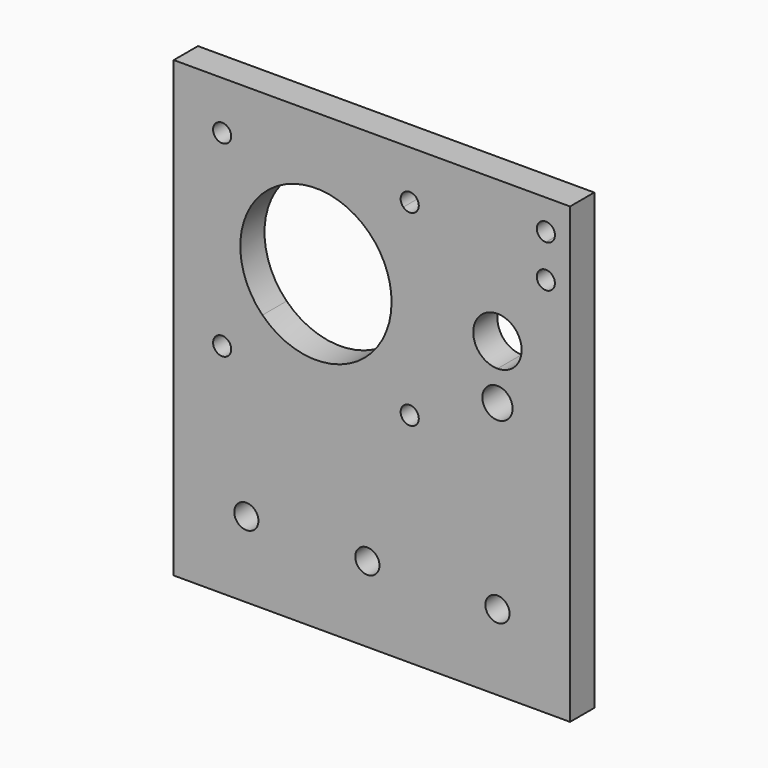
from build123d import *

# Parameters (mm, degrees)
F0_W     = 47
F0_H     = 50
F0_R     = 1.5
F1_DEPTH = 5


# Not quite as in the source:
# - a feature names something its author has since deleted; it is built from what else it names


with BuildPart() as f1:
    # F0 (on Front) → F1 (new body)
    with BuildSketch(Plane.XZ):
        with Locations((23.5, 25)):
            Rectangle(F0_W, F0_H)
        with BuildLine():
            ThreePointArc((9.5, 11), (6.6141807012, 10.4259748515), (9.0606601718, 12.0606601718))
            ThreePointArc((9.0606601718, 12.0606601718), (9.3858192988, 11.5740251485), (9.5, 11))
        make_face(mode=Mode.SUBTRACT)
        with Locations((39, 11)):
            Circle(F0_R, mode=Mode.SUBTRACT)
        with BuildLine():
            ThreePointArc((14.6611652352, 17.6611652352), (14.6611652352, 35.3388347648), (32.3388347648, 35.3388347648))
            ThreePointArc((32.3388347648, 35.3388347648), (35.0484941564, 31.2835429046), (36, 26.5))
            ThreePointArc((36, 26.5), (28.2835429046, 14.9515058436), (14.6611652352, 17.6611652352))
        make_face(mode=Mode.SUBTRACT)
        with Locations((8, 42)):
            Circle(F0_R, mode=Mode.SUBTRACT)
        with BuildLine():
            ThreePointArc((37.9393398282, 40.9393398282), (38.4259748515, 43.3858192988), (40.5, 42))
            ThreePointArc((40.5, 42), (39.5740251485, 40.6141807012), (37.9393398282, 40.9393398282))
        make_face(mode=Mode.SUBTRACT)
        with BuildLine():
            Line((47, 50), (47, 0))
            Line((47, 0), (47, -12.5))
            Line((47, -12.5), (51.5, -12.5))
            ThreePointArc((51.5, -12.5), (53.5, -10.5), (55.5, -12.5))
            Line((55.5, -12.5), (65.5, -12.5))
            Line((65.5, -12.5), (65.5, 26.5))
            Line((65.5, 26.5), (65.5, 50))
            Line((65.5, 50), (61.5, 50))
            Line((61.5, 50), (47, 50))
        make_face()
        with BuildLine():
            ThreePointArc((56, 17.5), (51.732233047, 15.732233047), (53.5, 20))
            ThreePointArc((53.5, 20), (55.267766953, 19.267766953), (56, 17.5))
        make_face(mode=Mode.SUBTRACT)
        with BuildLine():
            ThreePointArc((53.5, 22.5), (50.6715728753, 29.3284271247), (57.5, 26.5))
            ThreePointArc((57.5, 26.5), (56.3284271247, 23.6715728753), (53.5, 22.5))
        make_face(mode=Mode.SUBTRACT)
        with BuildLine():
            ThreePointArc((63, 38), (60.4393398282, 36.9393398282), (61.5, 39.5))
            ThreePointArc((61.5, 39.5), (62.5606601718, 39.0606601718), (63, 38))
        make_face(mode=Mode.SUBTRACT)
        with BuildLine():
            ThreePointArc((61.5, 43.5), (60, 45), (61.5, 46.5))
            ThreePointArc((61.5, 46.5), (62.5606601718, 46.0606601718), (63, 45))
            ThreePointArc((63, 45), (62.5606601718, 43.9393398282), (61.5, 43.5))
        make_face(mode=Mode.SUBTRACT)
        with BuildLine():
            Line((47, 0), (0, 0))
            Line((0, 0), (0, -12.5))
            Line((0, -12.5), (10, -12.5))
            ThreePointArc((10, -12.5), (12, -10.5), (14, -12.5))
            Line((14, -12.5), (30, -12.5))
            ThreePointArc((30, -12.5), (32, -10.5), (34, -12.5))
            Line((34, -12.5), (47, -12.5))
            Line((47, -12.5), (47, 0))
        make_face()
        with BuildLine():
            Line((10, -12.5), (0, -12.5))
            Line((0, -12.5), (0, -25))
            Line((0, -25), (47, -25))
            Line((47, -25), (47, -12.5))
            Line((47, -12.5), (34, -12.5))
            ThreePointArc((34, -12.5), (32, -14.5), (30, -12.5))
            Line((30, -12.5), (14, -12.5))
            ThreePointArc((14, -12.5), (12, -14.5), (10, -12.5))
        make_face()
        with BuildLine():
            Line((51.5, -12.5), (47, -12.5))
            Line((47, -12.5), (47, -25))
            Line((47, -25), (65.5, -25))
            Line((65.5, -25), (65.5, -12.5))
            Line((65.5, -12.5), (55.5, -12.5))
            ThreePointArc((55.5, -12.5), (53.5, -14.5), (51.5, -12.5))
        make_face()
    extrude(amount=F1_DEPTH)


solid = f1.part
